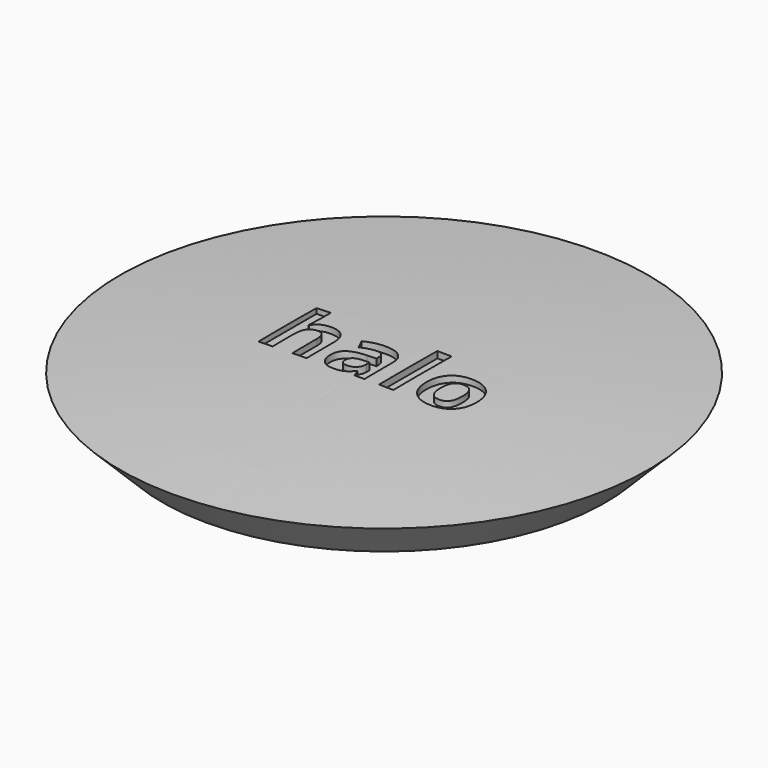
from build123d import *

# Parameters (mm, degrees)
F3_TEXT_SIZE = 4.5341834927
F4_DEPTH     = 27.8


# Not quite as in the source:
# - Text() gives the source's letters only with a copy of the font that has no kerning and outlines rounded to 1/6400 em; it was checked with that copy


with BuildPart() as f1:
    # F0 (on Right) → F1 (revolve)
    with BuildSketch(Plane.YZ):
        with BuildLine():
            Line((-10.5, 0), (0, 0))
            Line((0, 0), (0, 2.5217407112))
            ThreePointArc((0, 2.5217407112), (-6.2554418983, 2.3912487729), (-12.5, 2))
            Line((-12.5, 2), (-10.5, 0))
        make_face()
    revolve(axis=Axis((0, 0, 1.2608703556), (0, 0, -1)))

    # F3 (on offset) → F4 (cut)
    with BuildSketch(Plane.XY.offset(30)):
        with Locations((-5, -1.6323060574)):
            Text('halo', F3_TEXT_SIZE, font='Open Sans', font_style=FontStyle.BOLD, text_align=(TextAlign.LEFT, TextAlign.BOTTOM))
    extrude(amount=-F4_DEPTH, mode=Mode.SUBTRACT)


solid = f1.part
